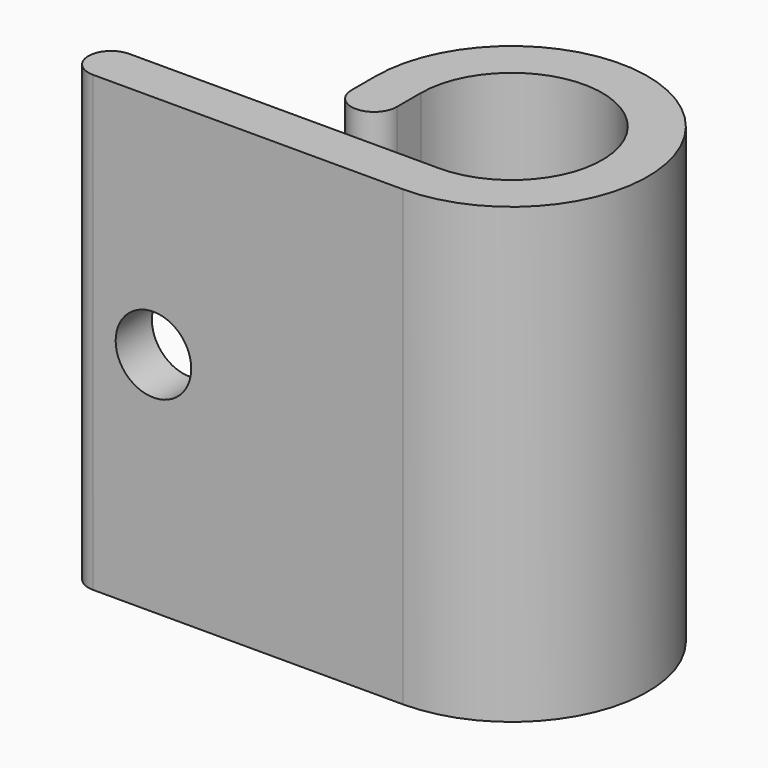
from build123d import *

# Parameters (mm, degrees)
F1_DEPTH = 15
F2_R     = 0.74999
F3_R     = 1.25
F4_DEPTH = 8.2


# Not quite as in the source:
# - a fillet or chamfer is up to 0.001 mm smaller than in the source, because OpenCascade refuses the exact size


with BuildPart() as f1:
    # F0 (on Top) → F1 (new body)
    with BuildSketch(Plane.XY):
        with BuildLine():
            ThreePointArc((-3, 0), (2.1213203436, 2.1213203436), (0, -3))
            Line((0, -3), (-11, -3))
            Line((-11, -3), (-11, -4.5))
            Line((-11, -4.5), (0, -4.5))
            ThreePointArc((0, -4.5), (3.1819805153, 3.1819805153), (-4.5, 0))
            Line((-4.5, 0), (-4.5, -1))
            ThreePointArc((-4.5, -1), (-3.75, -1.75), (-3, -1))
            Line((-3, -1), (-3, 0))
        make_face()
    extrude(amount=F1_DEPTH)

    # F2 (radius 0.75 in the source; OpenCascade refuses exactly that, so slightly less here)
    f2_edges = [f1.edges().sort_by_distance(p)[0] for p in [
        (-11, -3, 7.5),
        (-11, -4.5, 7.5),
    ]]
    fillet(f2_edges, radius=F2_R)

    # F3 (on face) → F4 (cut)
    with BuildSketch(Plane(origin=(0, -3, 0), x_dir=(-1, 0, 0), z_dir=(0, 1, 0))):
        with Locations((8.25, 7.5)):
            Circle(F3_R)
    extrude(amount=-F4_DEPTH, mode=Mode.SUBTRACT)


solid = f1.part
